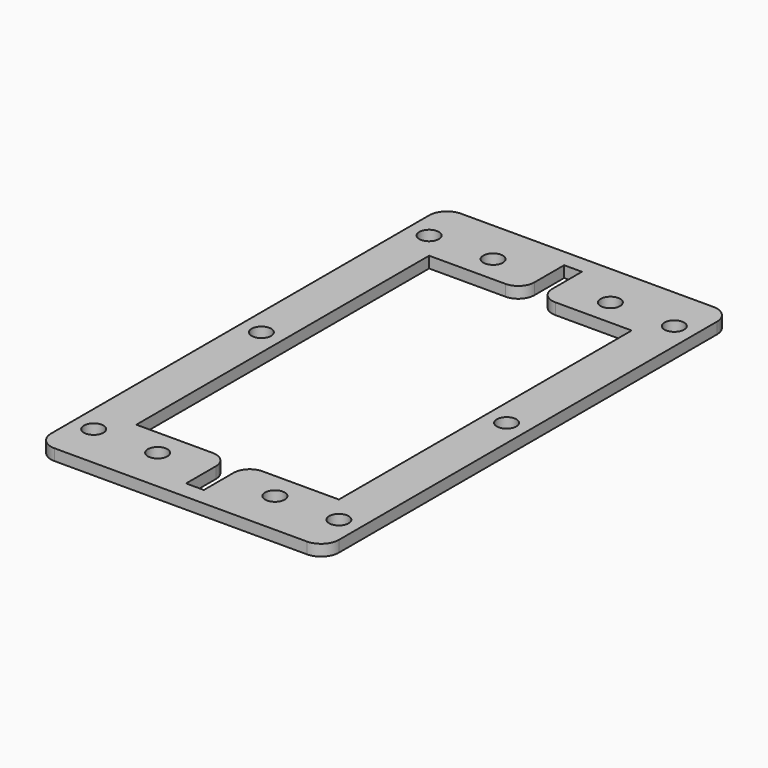
from build123d import *

# Parameters (mm, degrees)
F0_R     = 2.75
F1_DEPTH = 3.175


# Not quite as in the source:
# - a length typed as a fraction of an inch, garbled in the dataset ("3 / 203.2 mm" for 3/8 in), is restored


with BuildPart() as f1:
    # F0 (on Top) → F1 (new body)
    with BuildSketch(Plane.XY):
        with BuildLine():
            Line((-35.5, -71.5), (35.5, -71.5))
            ThreePointArc((35.5, -71.5), (39.0355339059, -70.0355339059), (40.5, -66.5))
            Line((40.5, -66.5), (40.5, 66.5))
            ThreePointArc((40.5, 66.5), (39.0355339059, 70.0355339059), (35.5, 71.5))
            Line((35.5, 71.5), (-35.5, 71.5))
            ThreePointArc((-35.5, 71.5), (-39.0355339059, 70.0355339059), (-40.5, 66.5))
            Line((-40.5, 66.5), (-40.5, -66.5))
            ThreePointArc((-40.5, -66.5), (-39.0355339059, -70.0355339059), (-35.5, -71.5))
        make_face()
        with Locations((-34.5, -59)):
            Circle(F0_R, mode=Mode.SUBTRACT)
        with Locations((-16.5, -59)):
            Circle(F0_R, mode=Mode.SUBTRACT)
        with Locations((16.5, -59)):
            Circle(F0_R, mode=Mode.SUBTRACT)
        with Locations((34.5, -59)):
            Circle(F0_R, mode=Mode.SUBTRACT)
        with Locations((-34.5, 0)):
            Circle(F0_R, mode=Mode.SUBTRACT)
        with Locations((-34.5, 59)):
            Circle(F0_R, mode=Mode.SUBTRACT)
        with Locations((-16.5, 59)):
            Circle(F0_R, mode=Mode.SUBTRACT)
        with BuildLine():
            Line((28.5, 51.5), (28.5, -51.5))
            Line((28.5, -51.5), (7, -51.5))
            ThreePointArc((7, -51.5), (3.8180194847, -52.8180194847), (2.5, -56))
            Line((2.5, -56), (2.5, -66.5))
            Line((2.5, -66.5), (-2.5, -66.5))
            Line((-2.5, -66.5), (-2.5, -56))
            ThreePointArc((-2.5, -56), (-3.8180194847, -52.8180194847), (-7, -51.5))
            Line((-7, -51.5), (-28.5, -51.5))
            Line((-28.5, -51.5), (-28.5, 51.5))
            Line((-28.5, 51.5), (-7, 51.5))
            ThreePointArc((-7, 51.5), (-3.8180194847, 52.8180194847), (-2.5, 56))
            Line((-2.5, 56), (-2.5, 66.5))
            Line((-2.5, 66.5), (2.5, 66.5))
            Line((2.5, 66.5), (2.5, 56))
            ThreePointArc((2.5, 56), (3.8180194847, 52.8180194847), (7, 51.5))
            Line((7, 51.5), (28.5, 51.5))
        make_face(mode=Mode.SUBTRACT)
        with Locations((34.5, 0)):
            Circle(F0_R, mode=Mode.SUBTRACT)
        with Locations((16.5, 59)):
            Circle(F0_R, mode=Mode.SUBTRACT)
        with Locations((34.5, 59)):
            Circle(F0_R, mode=Mode.SUBTRACT)
    extrude(amount=F1_DEPTH)


solid = f1.part
